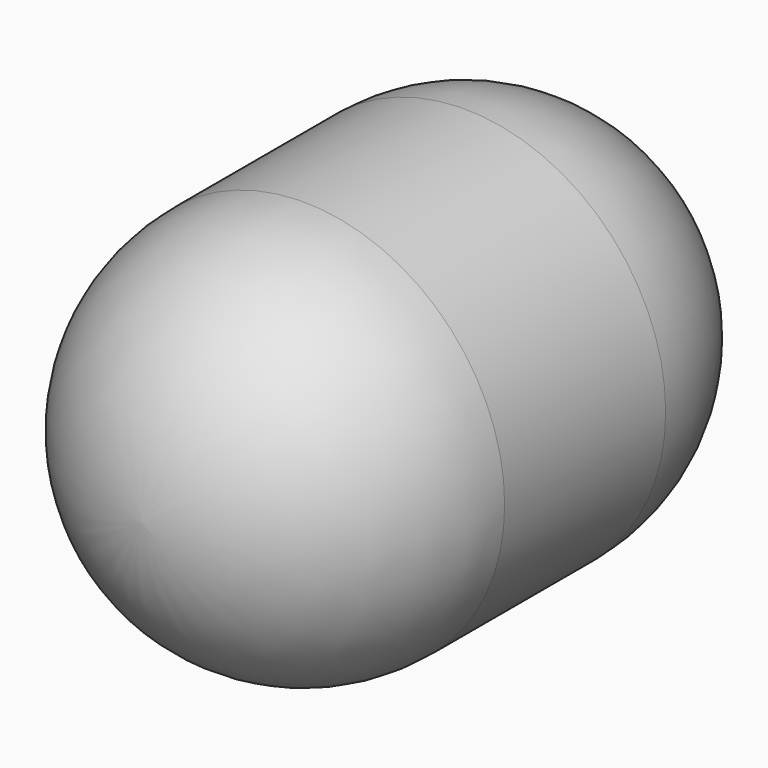
from build123d import *

# Parameters (mm, degrees)
F0_R          = 25.4
F1_DEPTH      = 50.8
F1_DEPTH_BACK = 25.4
F2_R          = 25.39999


# Not quite as in the source:
# - a fillet or chamfer is up to 0.001 mm smaller than in the source, because OpenCascade refuses the exact size


with BuildPart() as f1:
    # F0 (on Front) → F1 (new body, two sides)
    with BuildSketch(Plane.XZ) as f1_sk:
        Circle(F0_R)
    extrude(amount=F1_DEPTH)
    extrude(f1_sk.sketch, amount=-F1_DEPTH_BACK)

    # F2 (radius 25.4 in the source; OpenCascade refuses exactly that, so slightly less here)
    f2_edges = [f1.edges().sort_by_distance(p)[0] for p in [
        (-25.4, 25.4, 0),
        (-25.4, -50.8, 0),
    ]]
    fillet(f2_edges, radius=F2_R)


solid = f1.part
